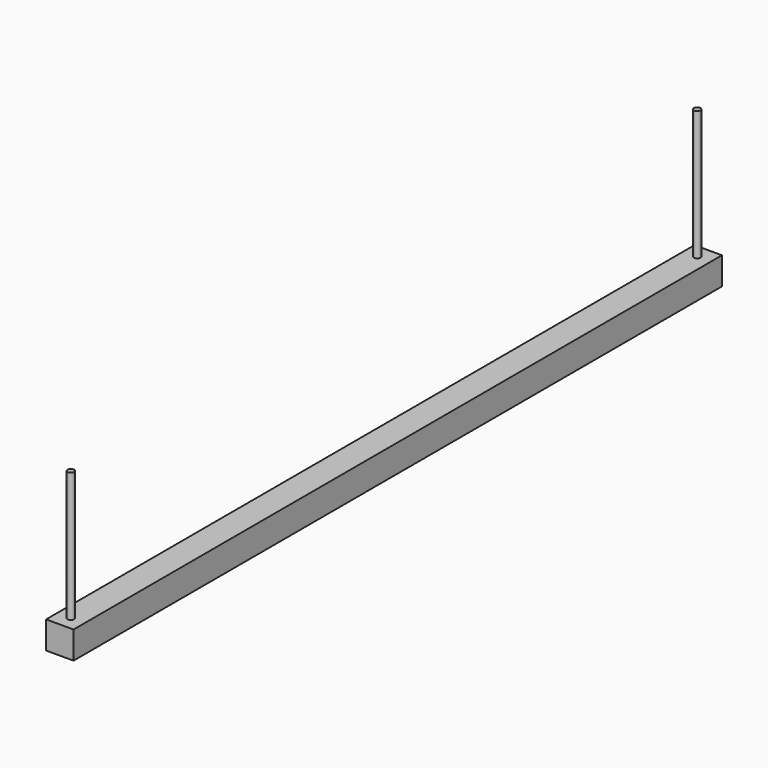
from build123d import *

# Parameters (mm, degrees)
F0_W     = 25.4
F0_H     = 25.4
F1_DEPTH = 375
F3_DEPTH = 375
F2_R     = 3
F4_DEPTH = 120


with BuildPart() as f1:
    # F0 (on Front) → F1 (new body, symmetric)
    with BuildSketch(Plane.XZ):
        Rectangle(F0_W, F0_H)
    extrude(amount=F1_DEPTH, both=True)

    # F2 (on face) → F4 (join)
    with BuildSketch(Plane.XY.offset(12.7)):
        with Locations((0, -362.3)):
            Circle(F2_R)
        with Locations((0, 362.3)):
            Circle(F2_R)
    extrude(amount=F4_DEPTH)


with BuildPart() as f3:
    # F0 (on Front) → F3 (new body, symmetric)
    with BuildSketch(Plane.XZ):
        Rectangle(F0_W, F0_H)
    extrude(amount=F3_DEPTH, both=True)


solid = Compound([f1.part, f3.part])
